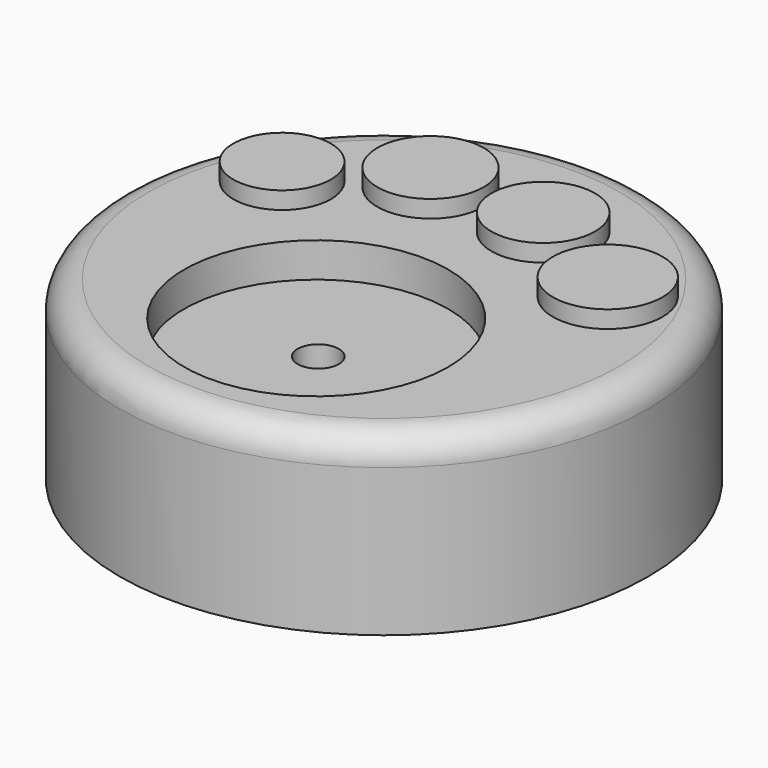
from build123d import *

# Parameters (mm, degrees)
F0_R      = 38.1
F2_DEPTH  = 25.4
F3_R      = 4.104163056
F4_R      = 7.676399804
F4_R_2    = 7.4730209118
F4_R_3    = 7.9111301116
F4_R_4    = 7.0349890874
F6_DEPTH  = 2.5
F7_R      = 19.05
F8_DEPTH  = 5
F9_R      = 5.715
F10_DEPTH = 3.9
F11_R     = 2.9751470693
F12_DEPTH = 24.001


# Not quite as in the source:
# - a feature names something its author has since deleted; it is built from what else it names


with BuildPart() as f2:
    # F0 (on Top) → F2 (new body)
    with BuildSketch(Plane.XY):
        with Locations((0, -4.1931332196)):
            Circle(F0_R)
    extrude(amount=F2_DEPTH)

    # F3
    f3_edges = [f2.edges().sort_by_distance(p)[0] for p in [
        (-38.1, -4.193133, 25.4),
    ]]
    fillet(f3_edges, radius=F3_R)

    # F4 (on face) → F6 (join)
    with BuildSketch(Plane.XY.offset(25.4)):
        with Locations((-9.9296038883, 16.6010573738)):
            Circle(F4_R)
        with Locations((6.8266042386, 15.9804562879)):
            Circle(F4_R_2)
        with Locations((22.3416063405, 8.2229533103)):
            Circle(F4_R_3)
        with Locations((-23.8931100186, 7.2920526448)):
            Circle(F4_R_4)
    extrude(amount=F6_DEPTH)

    # F7 (on face) → F8 (cut)
    with BuildSketch(Plane.XY.offset(25.4)):
        with Locations((0, -16.4202762372)):
            Circle(F7_R)
    extrude(amount=-F8_DEPTH, mode=Mode.SUBTRACT)

    # F9 (on face) → F10 (cut)
    with BuildSketch(Plane(origin=(0, 0, 0), x_dir=(1, 0, 0), z_dir=(0, 0, -1))):
        with Locations((0, 16.0560380752)):
            Circle(F9_R)
    extrude(amount=-F10_DEPTH, mode=Mode.SUBTRACT)

    # F11 (on face) → F12 (cut, through all)
    with BuildSketch(Plane(origin=(0, 0, 3.9), x_dir=(1, 0, 0), z_dir=(0, 0, -1))):
        with Locations((0, 16.0560380752)):
            Circle(F11_R)
    extrude(amount=-F12_DEPTH, mode=Mode.SUBTRACT)


solid = f2.part
